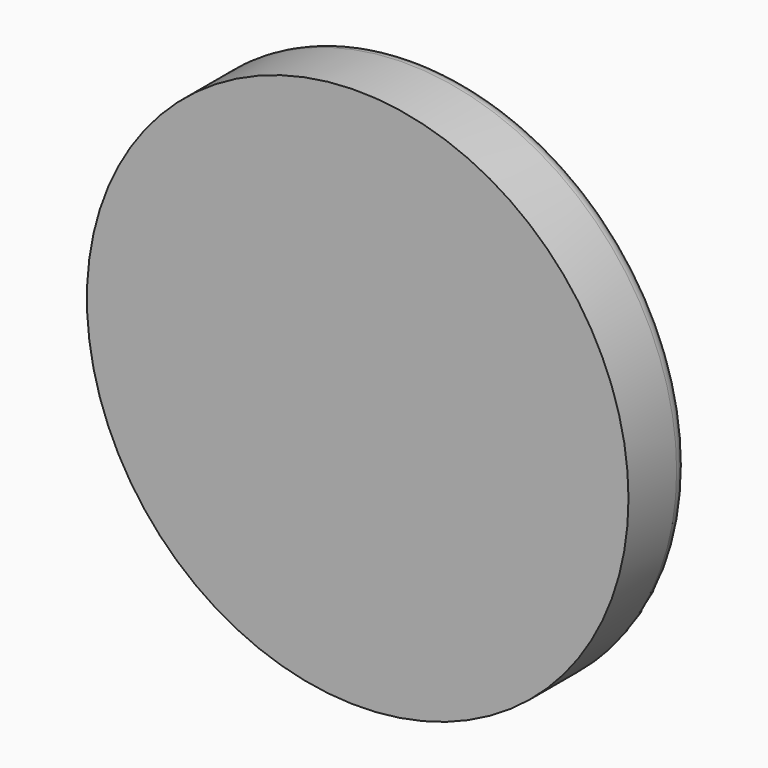
from build123d import *

# Parameters (mm, degrees)
F0_R     = 914.4
F1_DEPTH = 254
F2_R     = 50.8


# Not quite as in the source:
# - the program builds the solid bodies; features that only make, move or delete a surface that nothing else refers to are left out


with BuildPart() as f1:
    # F0 (on Front) → F1 (new body)
    with BuildSketch(Plane.XZ):
        Circle(F0_R)
    extrude(amount=-F1_DEPTH)

    # F2
    f2_edges = [f1.edges().sort_by_distance(p)[0] for p in [
        (-914.4, 254, 0),
    ]]
    fillet(f2_edges, radius=F2_R)


solid = f1.part
